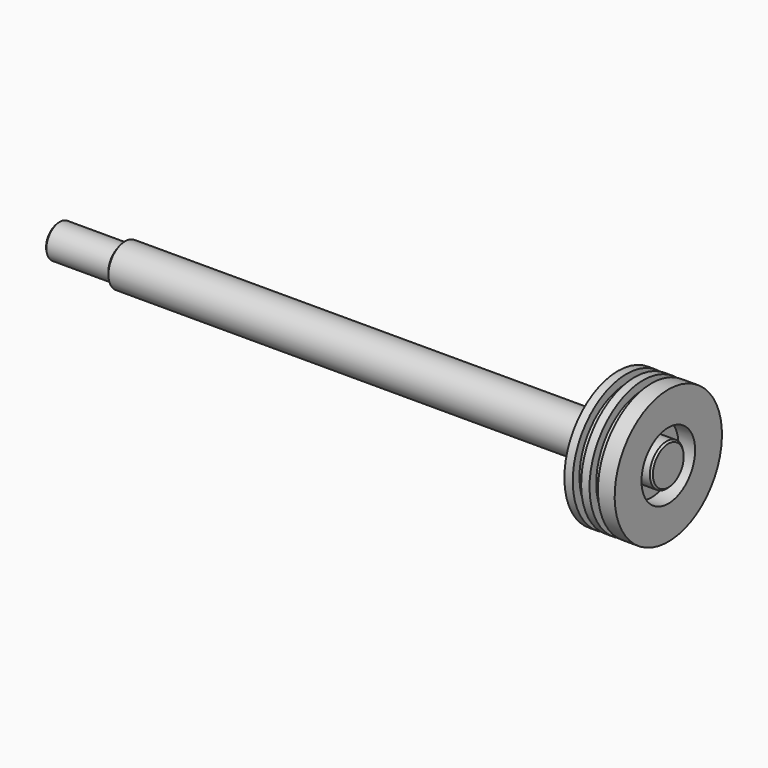
from build123d import *

# Parameters (mm, degrees)
F2_SIZE = 1
F3_SIZE = 1


# Not quite as in the source:
# - a feature names something its author has since deleted; it is built from what else it names


with BuildPart() as f1:
    # F0 (on Front) → F1 (revolve)
    with BuildSketch(Plane.XZ):
        Polygon((294, 12.5), (0, 12.5), (0, 7.5), (-2, 7.5), (-2, 10), (-40, 10), (-40, 0), (324, 0), (324, 12.5), (314, 12.5), (314, 20), (324, 20), (324, 40), (314, 40), (314, 35), (309, 35), (309, 40), (304, 40), (304, 35), (299, 35), (299, 40), (294, 40), align=None)
    revolve(axis=Axis((142, 0, 0), (1, 0, 0)))

    # F2
    f2_edges = [f1.edges().sort_by_distance(p)[0] for p in [
        (-2, 0, -7.5),
        (-40, 0, -10),
    ]]
    chamfer(f2_edges, length=F2_SIZE)

    # F3
    f3_edges = [f1.edges().sort_by_distance(p)[0] for p in [
        (324, 0, -12.5),
    ]]
    chamfer(f3_edges, length=F3_SIZE)


solid = f1.part
